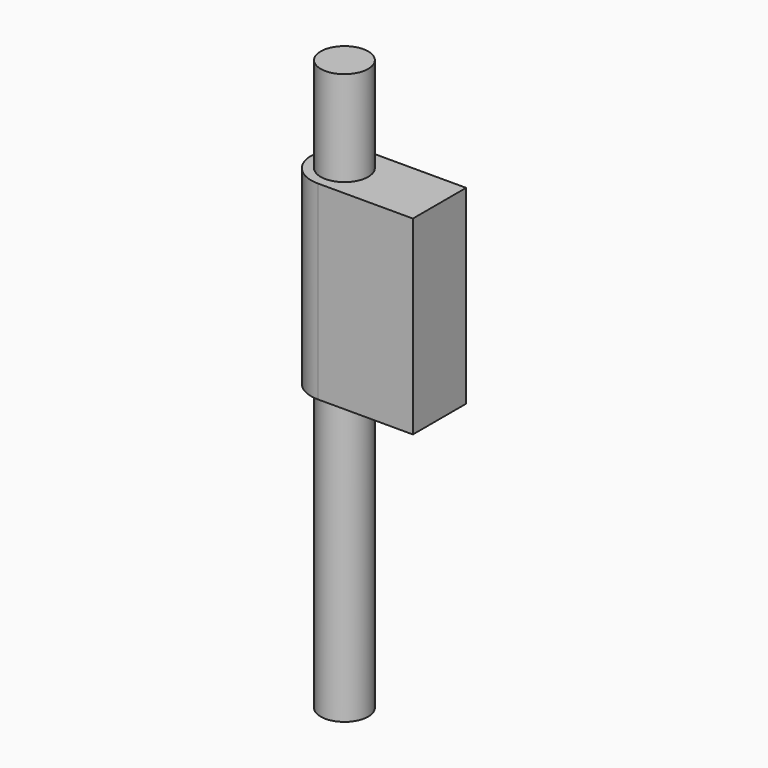
from build123d import *

# Parameters (mm, degrees)
F0_R     = 0.125
F1_DEPTH = 1
F2_DEPTH = 1.5


# Not quite as in the source:
# - ends of sketch curves that miss each other by under 0.0002 mm in the source are joined


with BuildPart() as f1:
    # F0 (on Top) → F1 (new body)
    with BuildSketch(Plane.XY):
        with BuildLine():
            Line((0.5, 0.175), (0, 0.175))
            ThreePointArc((0, 0.175), (-0.175, 0), (0, -0.175))
            Line((0, -0.175), (0.5, -0.175))
            Line((0.5, -0.175), (0.5, 0.175))
        make_face()
        Circle(F0_R, mode=Mode.SUBTRACT)
    extrude(amount=F1_DEPTH)


with BuildPart() as f2:
    # F0 (on Top) → F2 (new body, symmetric)
    with BuildSketch(Plane.XY):
        Circle(F0_R)
    extrude(amount=F2_DEPTH, both=True)


solid = Compound([f1.part, f2.part])
